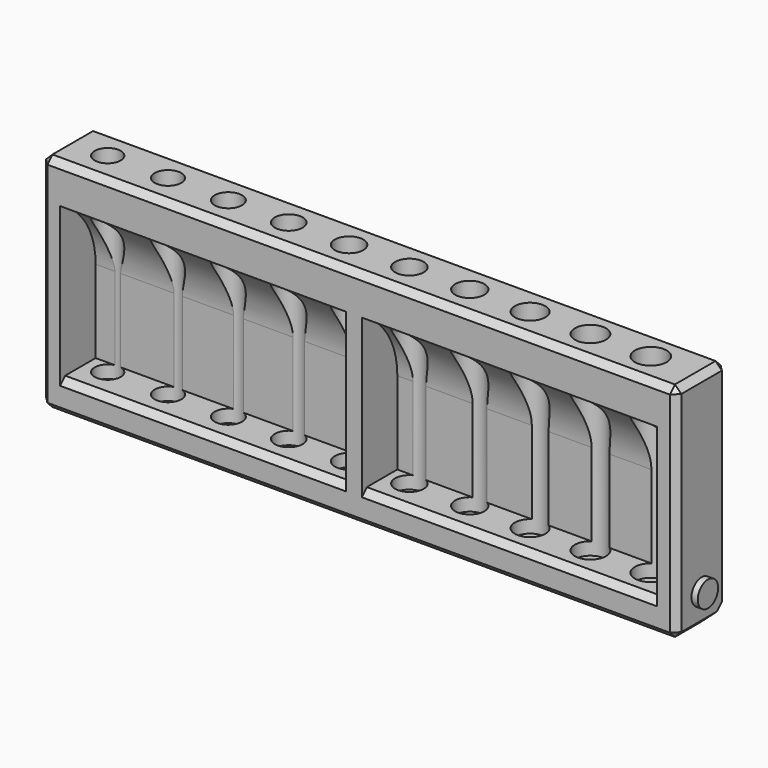
from build123d import *

# Parameters (mm, degrees)
F0_W          = 100
F0_H          = 10
F2_DEPTH      = 35
F3_START      = 3
F1_R          = 2.5
F1_R_2        = 2.45
F1_R_3        = 2.4
F1_R_4        = 2.3
F1_R_5        = 2.25
F1_R_6        = 2.2
F1_R_7        = 2.15
F1_R_8        = 2.1
F1_R_9        = 2.05
F3_DEPTH      = 37
F5_START      = -3
F5_DEPTH      = 46.5
F6_START      = -52
F6_DEPTH      = 45
F7_SIZE       = 1
F8_R          = 2
F9_DEPTH      = 2
F9_DEPTH_BACK = 1
F10_START     = -99
F10_DEPTH     = 2
F11_T1_DEPTH  = 123


# Not quite as in the source:
# - a fillet or chamfer that OpenCascade refuses, or shapes differently, is made with other operations: its cross-section is extruded or revolved along the edge and cut away or added


with BuildPart() as f2:
    # F0 (on Top) → F2 (new body)
    with BuildSketch(Plane.XY):
        with Locations((-50, -5)):
            Rectangle(F0_W, F0_H)
    extrude(amount=F2_DEPTH)

    # F1 (on Top) → F3 (cut)
    with BuildSketch(Plane.XY.offset(F3_START)):
        with Locations((-8, -5)):
            Circle(F1_R)
        with Locations((-17.5, -5)):
            Circle(F1_R_2)
        with Locations((-27, -5)):
            Circle(F1_R_3)
        with Locations((-36.5, -5)):
            Circle(F1_R_4)
        with Locations((-46, -5)):
            Circle(F1_R_5)
        with Locations((-55.5, -5)):
            Circle(F1_R_5)
        with Locations((-65, -5)):
            Circle(F1_R_6)
        with Locations((-74.5, -5)):
            Circle(F1_R_7)
        with Locations((-84, -5)):
            Circle(F1_R_8)
        with Locations((-93.5, -5)):
            Circle(F1_R_9)
    extrude(amount=F3_DEPTH, mode=Mode.SUBTRACT)

    # F4 (on Right) → F5 (cut)
    with BuildSketch(Plane.YZ.offset(F5_START)):
        with BuildLine():
            Line((-13, 29.8321595662), (-13, 5))
            Line((-13, 5), (-3, 5))
            Line((-3, 5), (-3, 18))
            ThreePointArc((-3, 18), (-5.8348486101, 25.7459666924), (-13, 29.8321595662))
        make_face()
        with BuildLine():
            ThreePointArc((-15, 30), (-13.9964848766, 29.9579662735), (-13, 29.8321595662))
            Line((-13, 29.8321595662), (-13, 30))
            Line((-13, 30), (-15, 30))
        make_face()
    extrude(amount=-F5_DEPTH, mode=Mode.SUBTRACT)

    # F4 (on Right) → F6 (cut)
    with BuildSketch(Plane.YZ.offset(F6_START)):
        with BuildLine():
            Line((-13, 29.8321595662), (-13, 5))
            Line((-13, 5), (-3, 5))
            Line((-3, 5), (-3, 18))
            ThreePointArc((-3, 18), (-5.8348486101, 25.7459666924), (-13, 29.8321595662))
        make_face()
        with BuildLine():
            ThreePointArc((-15, 30), (-13.9964848766, 29.9579662735), (-13, 29.8321595662))
            Line((-13, 29.8321595662), (-13, 30))
            Line((-13, 30), (-15, 30))
        make_face()
    extrude(amount=-F6_DEPTH, mode=Mode.SUBTRACT)

    # F7
    f7_edges = [f2.edges().sort_by_distance(p)[0] for p in [
        (-50, -10, 35),
        (-100, -5, 35),
        (-50, 0, 35),
        (0, -5, 35),
        (0, -10, 17.5),
        (0, 0, 17.5),
        (0, -5, 0),
        (-50, -10, 0),
        (-100, -10, 17.5),
        (-74.5, -10, 5),
        (-26.25, -10, 5),
        (-100, -5, 0),
        (-100, 0, 17.5),
    ]]
    chamfer(f7_edges, length=F7_SIZE)

    # F8 (on Right) → F9 (join, two sides)
    with BuildSketch(Plane.YZ) as f9_sk:
        with Locations((-5, 5)):
            Circle(F8_R)
    extrude(amount=-F9_DEPTH)
    extrude(f9_sk.sketch, amount=F9_DEPTH_BACK)

    # F8 (on Right) → F10 (join)
    with BuildSketch(Plane.YZ.offset(F10_START)):
        with Locations((-5, 5)):
            Circle(F8_R)
    extrude(amount=-F10_DEPTH)

    # F11: fillet of radius 5 on 1 edges, made by hand

    # F11_s2 → F11_t1 (cut)
    with BuildSketch(Plane.YZ.offset(-111.5)):
        with BuildLine():
            ThreePointArc((0, 5), (-1.4644660941, 1.4644660941), (-5, 0))
            Line((-5, 0), (0, 0))
            Line((0, 0), (0, 5))
        make_face()
    extrude(amount=F11_T1_DEPTH, mode=Mode.SUBTRACT)


solid = f2.part
